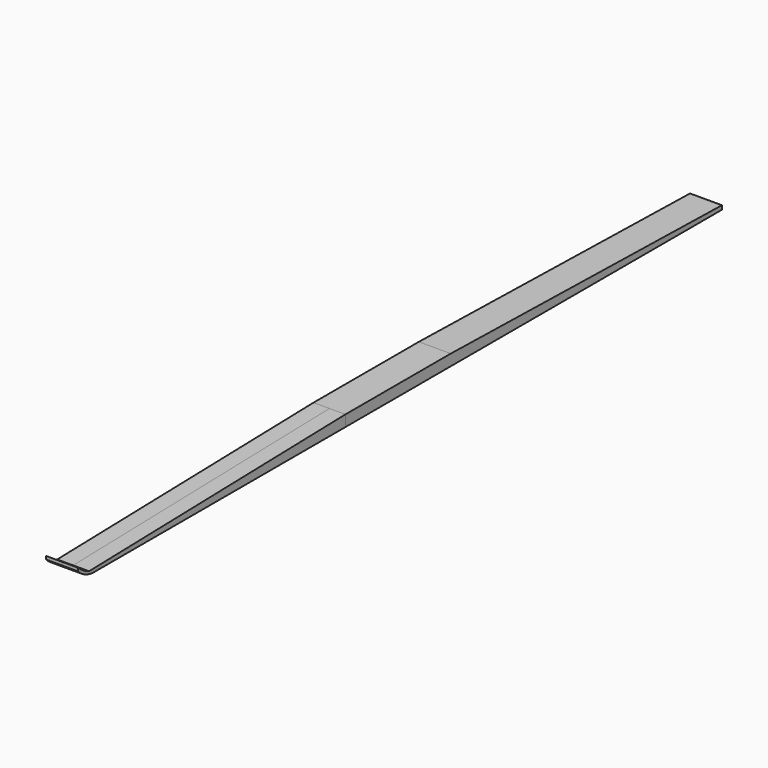
from build123d import *

# Parameters (mm, degrees)
F0_W     = 8
F0_H     = 2.8
F1_DEPTH = 16.5
F2_DEPTH = 16.5
F4_DEPTH = 4
F5_DEPTH = 4
F6_DEPTH = 4
F7_DEPTH = 4


# Not quite as in the source:
# - a feature names something its author has since deleted; it is built from what else it names


with BuildPart() as f1:
    # F0 (on Front) → F1 (new body)
    with BuildSketch(Plane.XZ):
        Rectangle(F0_W, F0_H)
    extrude(amount=F1_DEPTH)

    # F0 (on Front) → F2 (join)
    with BuildSketch(Plane.XZ):
        Rectangle(F0_W, F0_H)
    extrude(amount=-F2_DEPTH)

    # F3 (on Right) → F4 (join)
    with BuildSketch(Plane.YZ):
        Polygon((101.4993405342, -0.3997026253), (16.4993405342, 1.3993438333), (16.4993405342, -1.3997026253), (101.4993405342, -1.3997026253), align=None)
    extrude(amount=F4_DEPTH)

    # F3 (on Right) → F5 (join)
    with BuildSketch(Plane.YZ):
        Polygon((101.4993405342, -0.3997026253), (16.4993405342, 1.3993438333), (16.4993405342, -1.3997026253), (101.4993405342, -1.3997026253), align=None)
    extrude(amount=-F5_DEPTH)


with BuildPart() as f4:
    # F3 (on Right) → F4, piece 2 (new body)
    with BuildSketch(Plane.YZ):
        with BuildLine():
            Line((-94.7134718299, -1.3999422081), (-92.9198265076, -1.3999422081))
            ThreePointArc((-92.9198265076, -1.3999422081), (-94.9201368355, -1.1517222137), (-96.8468752203, -0.5596632892))
            Line((-96.8468752203, -0.5596632892), (-98.4500434109, -0.5987649524))
            ThreePointArc((-98.4500434109, -0.5987649524), (-97.0768797518, -1.1494141491), (-95.618788992, -1.3999422081))
            Line((-95.618788992, -1.3999422081), (-94.7134718299, -1.3999422081))
        make_face()
    extrude(amount=F4_DEPTH)


with BuildPart() as f5:
    # F3 (on Right) → F5, piece 2 (new body)
    with BuildSketch(Plane.YZ):
        with BuildLine():
            Line((-94.7134718299, -1.3999422081), (-92.9198265076, -1.3999422081))
            ThreePointArc((-92.9198265076, -1.3999422081), (-94.9201368355, -1.1517222137), (-96.8468752203, -0.5596632892))
            Line((-96.8468752203, -0.5596632892), (-98.4500434109, -0.5987649524))
            ThreePointArc((-98.4500434109, -0.5987649524), (-97.0768797518, -1.1494141491), (-95.618788992, -1.3999422081))
            Line((-95.618788992, -1.3999422081), (-94.7134718299, -1.3999422081))
        make_face()
    extrude(amount=-F5_DEPTH)


with BuildPart() as f6:
    # F3 (on Right) → F6 (new body)
    with BuildSketch(Plane.YZ):
        with BuildLine():
            Line((-92.9198265076, -1.3999422081), (-16.4983108938, -1.3999422081))
            Line((-16.4983108938, -1.3999422081), (-16.4983108938, 1.4000577919))
            Line((-16.4983108938, 1.4000577919), (-96.8468752203, -0.5596632892))
            ThreePointArc((-96.8468752203, -0.5596632892), (-94.9201368355, -1.1517222137), (-92.9198265076, -1.3999422081))
        make_face()
        with BuildLine():
            Line((-98.4500434109, -0.5987649524), (-96.8468752203, -0.5596632892))
            ThreePointArc((-96.8468752203, -0.5596632892), (-98.6758535312, 0.3799035578), (-100.3093346953, 1.6287777741))
            Line((-100.3093346953, 1.6287777741), (-100.3093346953, 0.8287777741))
            ThreePointArc((-100.3093346953, 0.8287777741), (-99.4397174277, 0.036822948), (-98.4500434109, -0.5987649524))
        make_face()
        with BuildLine():
            Line((-94.7134718299, -1.3999422081), (-92.9198265076, -1.3999422081))
            ThreePointArc((-92.9198265076, -1.3999422081), (-94.9201368355, -1.1517222137), (-96.8468752203, -0.5596632892))
            Line((-96.8468752203, -0.5596632892), (-98.4500434109, -0.5987649524))
            ThreePointArc((-98.4500434109, -0.5987649524), (-97.0768797518, -1.1494141491), (-95.618788992, -1.3999422081))
            Line((-95.618788992, -1.3999422081), (-94.7134718299, -1.3999422081))
        make_face()
    extrude(amount=F6_DEPTH)


with BuildPart() as f7:
    # F3 (on Right) → F7 (new body)
    with BuildSketch(Plane.YZ):
        with BuildLine():
            Line((-92.9198265076, -1.3999422081), (-16.4983108938, -1.3999422081))
            Line((-16.4983108938, -1.3999422081), (-16.4983108938, 1.4000577919))
            Line((-16.4983108938, 1.4000577919), (-96.8468752203, -0.5596632892))
            ThreePointArc((-96.8468752203, -0.5596632892), (-94.9201368355, -1.1517222137), (-92.9198265076, -1.3999422081))
        make_face()
        with BuildLine():
            Line((-98.4500434109, -0.5987649524), (-96.8468752203, -0.5596632892))
            ThreePointArc((-96.8468752203, -0.5596632892), (-98.6758535312, 0.3799035578), (-100.3093346953, 1.6287777741))
            Line((-100.3093346953, 1.6287777741), (-100.3093346953, 0.8287777741))
            ThreePointArc((-100.3093346953, 0.8287777741), (-99.4397174277, 0.036822948), (-98.4500434109, -0.5987649524))
        make_face()
        with BuildLine():
            Line((-94.7134718299, -1.3999422081), (-92.9198265076, -1.3999422081))
            ThreePointArc((-92.9198265076, -1.3999422081), (-94.9201368355, -1.1517222137), (-96.8468752203, -0.5596632892))
            Line((-96.8468752203, -0.5596632892), (-98.4500434109, -0.5987649524))
            ThreePointArc((-98.4500434109, -0.5987649524), (-97.0768797518, -1.1494141491), (-95.618788992, -1.3999422081))
            Line((-95.618788992, -1.3999422081), (-94.7134718299, -1.3999422081))
        make_face()
    extrude(amount=-F7_DEPTH)


solid = Compound([f1.part, f4.part, f5.part, f6.part, f7.part])
